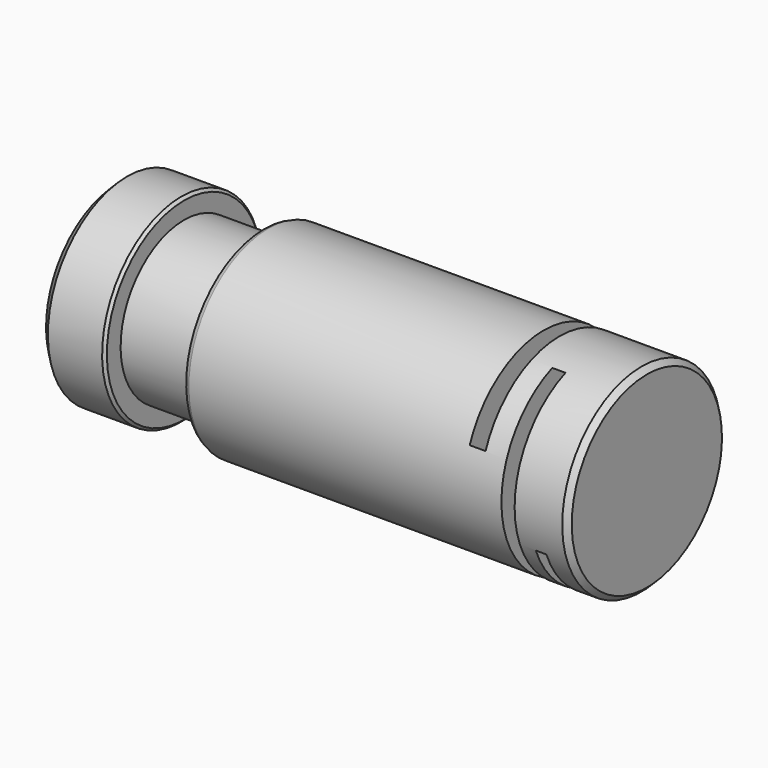
from build123d import *

# Parameters (mm, degrees)
F2_SIZE   = 0.7
F3_SIZE   = 0.2
F4_W      = 1
F4_H      = 14
F6_DEPTH  = 7.5
F7_W      = 1.2
F7_H      = 14
F8_DEPTH  = 7.5
F9_W      = 0.8
F9_H      = 14
F10_DEPTH = 7.5


# Not quite as in the source:
# - a fillet or chamfer that OpenCascade refuses, or shapes differently, is made with other operations: its cross-section is extruded or revolved along the edge and cut away or added


with BuildPart() as f1:
    # F0 (on Front) → F1 (revolve)
    with BuildSketch(Plane.XZ):
        Polygon((0, 7.5), (0, 0), (40, 0), (40, 7.5), (11, 7.5), (11, 6), (5, 6), (5, 7.5), align=None)
    revolve(axis=Axis((20, 0, 0), (1, 0, 0)))

    # F2
    f2_edges = [f1.edges().sort_by_distance(p)[0] for p in [
        (0, 0, -7.5),
    ]]
    chamfer(f2_edges, length=F2_SIZE)

    # F3
    f3_edges = [f1.edges().sort_by_distance(p)[0] for p in [
        (5, 0, -7.5),
        (11, 0, -7.5),
    ]]
    chamfer(f3_edges, length=F3_SIZE)

    # F5: chamfer of 0.4 on 3 edges, made by hand

    # F5_s1 → F5_t2 (revolve, cut)
    with BuildSketch(Plane.XZ):
        Polygon((11.0828427125, 7.3828427125), (11.3656854249, 7.5), (11.2, 7.5), align=None)
    revolve(axis=Axis((11.2, 0, 0), (1, 0, 0)), mode=Mode.SUBTRACT)

    # F5_s3 → F5_t4 (revolve, cut)
    with BuildSketch(Plane.XZ):
        Polygon((39.6, 7.5), (40, 7.1), (40, 7.5), align=None)
    revolve(axis=Axis((40, 0, 0), (1, 0, 0)), mode=Mode.SUBTRACT)

    # F4 (on Front) → F6 (cut)
    with BuildSketch(Plane.XZ):
        with Locations((35.5, 0)):
            Rectangle(F4_W, F4_H)
    extrude(amount=F6_DEPTH, mode=Mode.SUBTRACT)

    # F7 (on Top) → F8 (cut)
    with BuildSketch(Plane.XY):
        with Locations((32.8, 0)):
            Rectangle(F7_W, F7_H)
    extrude(amount=F8_DEPTH, mode=Mode.SUBTRACT)

    # F9 (on Top) → F10 (cut)
    with BuildSketch(Plane.XY):
        with Locations((37.6, 0)):
            Rectangle(F9_W, F9_H)
    extrude(amount=-F10_DEPTH, mode=Mode.SUBTRACT)


solid = f1.part
